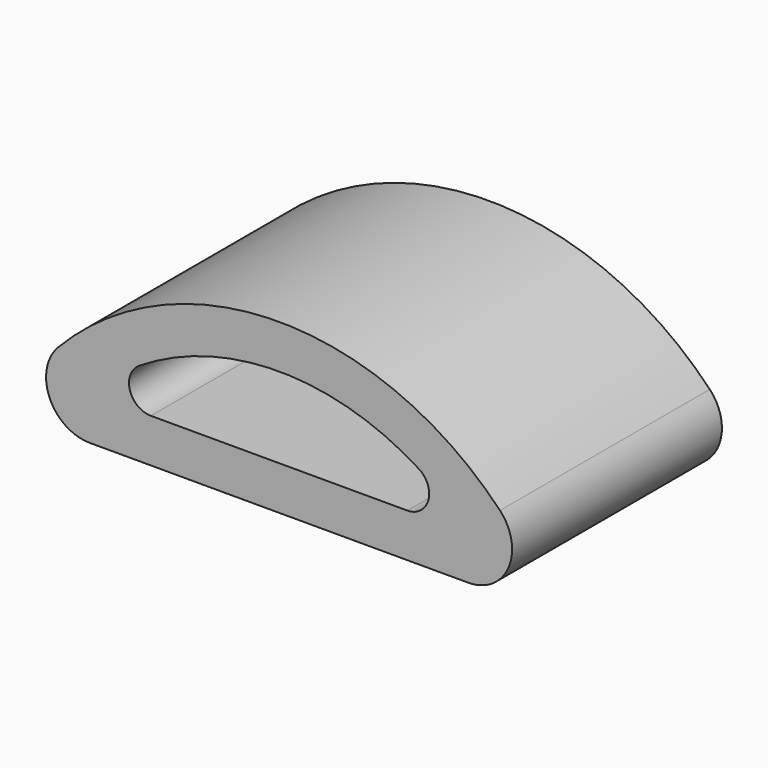
from build123d import *

# Parameters (mm, degrees)
F1_DEPTH = 12
F2_T     = -2
F3_R     = 2
F4_R     = 1


# Not quite as in the source:
# - a feature of the source that left no trace in its solid (it failed there, or was rolled back) is left out


with BuildPart() as f1:
    # F0 (on Front) → F1 (new body)
    with BuildSketch(Plane.XZ):
        with BuildLine():
            Line((-12.5, 0), (12.5, 0))
            ThreePointArc((12.5, 0), (0, 7.6952398935), (-12.5, 0))
        make_face()
    extrude(amount=F1_DEPTH)

    # F2
    f2_openings = [f1.faces().sort_by_distance(p)[0] for p in [
        (0, -12, 3.164528),
        (0, 0, 3.164528),
    ]]
    offset(amount=F2_T, openings=f2_openings)

    # F3
    f3_edges = [f1.edges().sort_by_distance(p)[0] for p in [
        (12.5, -6, 0),
        (-12.5, -6, 0),
    ]]
    fillet(f3_edges, radius=F3_R)

    # F4
    f4_edges = [f1.edges().sort_by_distance(p)[0] for p in [
        (-8.662041, -6, 2),
        (8.662041, -6, 2),
    ]]
    fillet(f4_edges, radius=F4_R)


solid = f1.part
